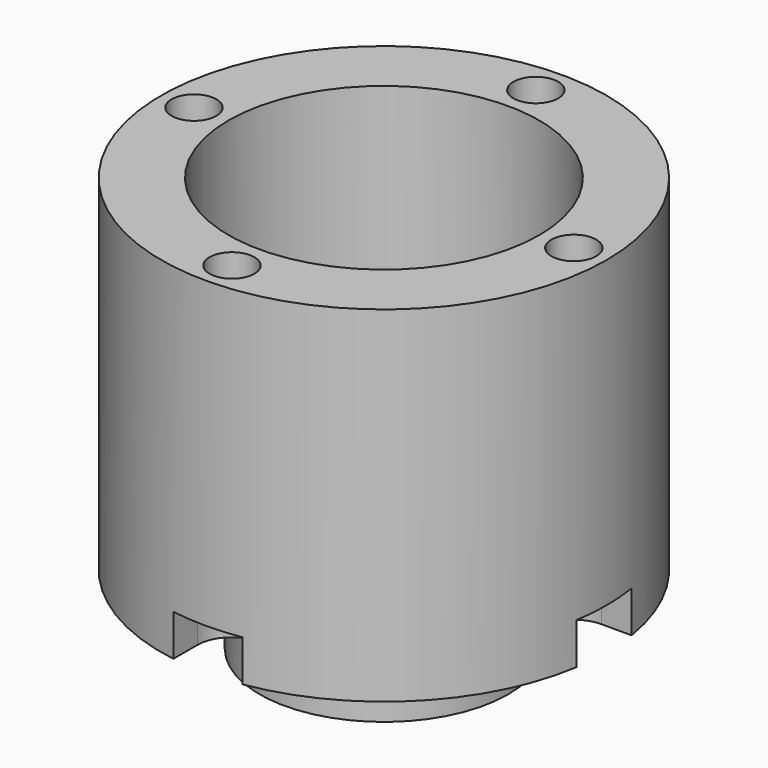
from build123d import *

# Parameters (mm, degrees)
F0_R            = 32.25
F1_DEPTH        = 50
F2_R            = 22.5
F3_DEPTH        = 40
F4_R            = 18
F5_DEPTH        = 10
F7_DEPTH        = 6
F7_COPIES_COUNT = 4
F8_D            = 6.5
F8_COPIES_COUNT = 4
F10_D           = 4
F11_D           = 6.8
F11_DEPTH       = 17
F11_TIP         = 2.0429261047
F12_D           = 6.8
F12_DEPTH       = 7
F12_TIP         = 2.0429261047
F14_D           = 6.8
F14_DEPTH       = 11
F14_TIP         = 2.0429261047


# Not quite as in the source:
# - a pattern or mirror of a feature is missing from the dataset's text; its kind, count and spacing are read off the source's solid


with BuildPart() as f1:
    # F0 (on Top) → F1 (new body)
    with BuildSketch(Plane.XY):
        Circle(F0_R)
    extrude(amount=F1_DEPTH)

    # F2 (on face) → F3 (cut)
    with BuildSketch(Plane.XY.offset(50)):
        Circle(F2_R)
    extrude(amount=-F3_DEPTH, mode=Mode.SUBTRACT)

    # F4 (on Top) → F5 (join)
    with BuildSketch(Plane.XY):
        Circle(F4_R)
    extrude(amount=-F5_DEPTH)

    # F6 (on Top) → F7 (cut)
    with BuildSketch(Plane.XY):
        with BuildLine():
            Line((-35, -5), (-27.5, -5))
            ThreePointArc((-27.5, -5), (-22.5, 0), (-27.5, 5))
            Line((-27.5, 5), (-35, 5))
            Line((-35, 5), (-35, -5))
        make_face()
    f7 = extrude(amount=F7_DEPTH, mode=Mode.SUBTRACT)

    # F7_copies: F7 ×4 about axis
    f7_copies_axis = Axis((0, 0, 0), (0, 0, 1))
    for i in range(1, F7_COPIES_COUNT):
        add(f7.rotate(f7_copies_axis, i * 360 / F7_COPIES_COUNT), mode=Mode.SUBTRACT)

    # F8 (through all)
    with Locations(Plane(origin=(0, 0, 0), x_dir=(1, 0, 0), z_dir=(0, 0, -1))):
        with Locations((-27.5, 0)):
            f8 = Hole(F8_D / 2)

    # F8_copies: F8 ×4 about axis
    f8_copies_axis = Axis((0, 0, 0), (0, 0, 1))
    for i in range(1, F8_COPIES_COUNT):
        add(f8.rotate(f8_copies_axis, i * 360 / F8_COPIES_COUNT), mode=Mode.SUBTRACT)

    # F10 (through all)
    with Locations(Plane(origin=(0, 0, -10), x_dir=(1, 0, 0), z_dir=(0, 0, -1))):
        with Locations((-10, 0), (10, 0)):
            Hole(F10_D / 2)

    # F11
    with Locations(Plane(origin=(0, 0, -10), x_dir=(1, 0, 0), z_dir=(0, 0, -1))):
        with Locations((-10, 0)):
            Hole(F11_D / 2, depth=F11_DEPTH)
            with Locations((0, 0, -(F11_DEPTH + F11_TIP / 2))):  # 118° drill point
                Cone(0, F11_D / 2, F11_TIP, mode=Mode.SUBTRACT)

    # F12
    with Locations(Plane(origin=(0, 0, -10), x_dir=(1, 0, 0), z_dir=(0, 0, -1))):
        with Locations((10, 0)):
            Hole(F12_D / 2, depth=F12_DEPTH)
            with Locations((0, 0, -(F12_DEPTH + F12_TIP / 2))):  # 118° drill point
                Cone(0, F12_D / 2, F12_TIP, mode=Mode.SUBTRACT)

    # F14
    with Locations(Plane.XY.offset(10)):
        with Locations((10, 0)):
            Hole(F14_D / 2, depth=F14_DEPTH)
            with Locations((0, 0, -(F14_DEPTH + F14_TIP / 2))):  # 118° drill point
                Cone(0, F14_D / 2, F14_TIP, mode=Mode.SUBTRACT)


solid = f1.part
